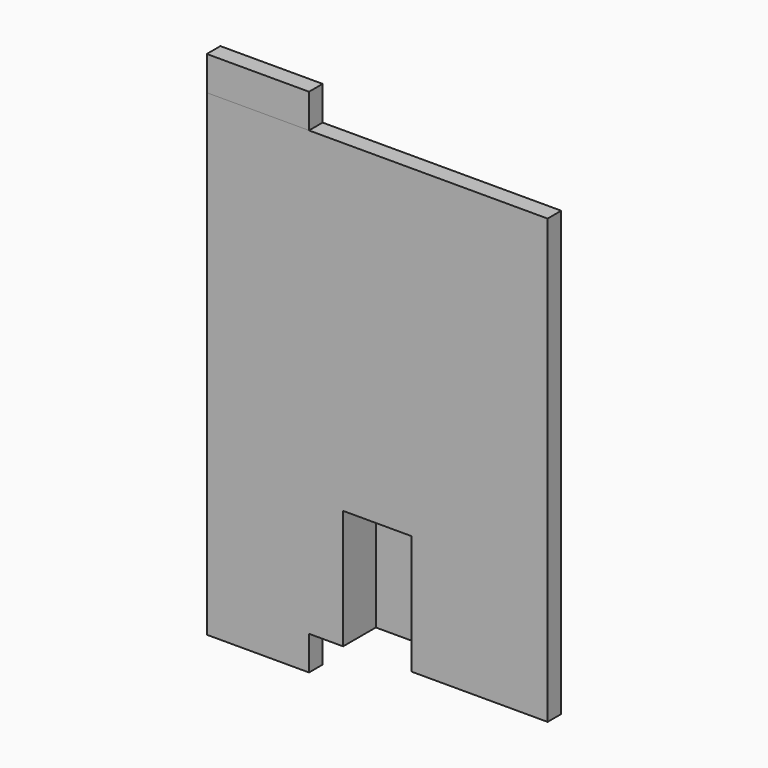
from build123d import *

# Parameters (mm, degrees)
F0_W      = 127
F0_H      = 165.1
F1_DEPTH  = 6.35
F2_W      = 12.7
F2_H      = 44.45
F3_DEPTH  = 25.4
F4_DEPTH  = 19.05
F5_W      = 25.4
F5_H      = 3.81
F6_DEPTH  = 44.45
F7_W      = 38.1
F7_H      = 12.7
F8_DEPTH  = 6.35
F9_W      = 38.1
F9_H      = 8.89
F10_DEPTH = 2.54
F11_W     = 38.1
F11_H     = 12.7
F12_DEPTH = 6.35


# Not quite as in the source:
# - a length typed as a fraction of an inch, garbled in the dataset ("3 / 203.2 mm" for 3/8 in), is restored


with BuildPart() as f1:
    # F0 (on Front) → F1 (new body)
    with BuildSketch(Plane.XZ):
        with Locations((10.689943251, 15.6320472565)):
            Rectangle(F0_W, F0_H)
    extrude(amount=F1_DEPTH)

    # F2 (on face) → F3 (cut)
    with BuildSketch(Plane.XZ.offset(6.35)):
        with Locations((4.339943251, -44.6929527435)):
            Rectangle(F2_W, F2_H)
        with Locations((17.039943251, -44.6929527435)):
            Rectangle(F2_W, F2_H)
    extrude(amount=-F3_DEPTH, mode=Mode.SUBTRACT)

    # F2 (on face) → F4 (join)
    with BuildSketch(Plane.XZ.offset(6.35)):
        Polygon((10.689943251, -22.4679527435), (10.689943251, -18.6579527435), (-5.820056749, -18.6579527435), (-5.820056749, -66.9179527435), (-2.010056749, -66.9179527435), (-2.010056749, -22.4679527435), align=None)
        Polygon((27.199943251, -18.6579527435), (10.689943251, -18.6579527435), (10.689943251, -22.4679527435), (23.389943251, -22.4679527435), (23.389943251, -66.9179527435), (27.199943251, -66.9179527435), align=None)
    extrude(amount=-F4_DEPTH)

    # F5 (on face) → F6 (join)
    with BuildSketch(Plane(origin=(0, 0, -22.4679527435), x_dir=(1, 0, 0), z_dir=(0, 0, -1))):
        with Locations((10.689943251, -10.795)):
            Rectangle(F5_W, F5_H)
    extrude(amount=F6_DEPTH)

    # F11 (on face) → F12 (join)
    with BuildSketch(Plane.XZ.offset(6.35)):
        with Locations((-33.760056749, -73.2679527435)):
            Rectangle(F11_W, F11_H)
    extrude(amount=-F12_DEPTH)


with BuildPart() as f8:
    # F7 (on face) → F8 (new body)
    with BuildSketch(Plane.XZ.offset(6.35)):
        with Locations((-33.760056749, 104.5320472565)):
            Rectangle(F7_W, F7_H)
    extrude(amount=-F8_DEPTH)


with BuildPart() as f10:
    # F9 (on face) → F10 (new body)
    with BuildSketch(Plane.XZ.offset(6.35)):
        with Locations((-33.760056749, 110.6541514468)):
            Rectangle(F9_W, F9_H)
    extrude(amount=F10_DEPTH)


solid = Compound([f1.part, f8.part])
